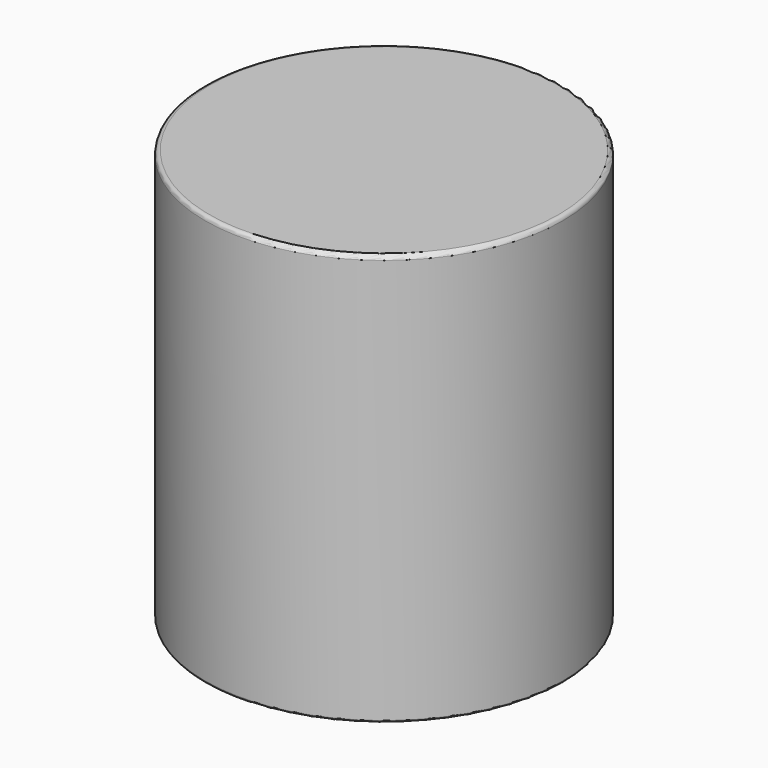
from build123d import *

# Parameters (mm, degrees)
F0_R     = 43.5
F0_R_2   = 42.5
F1_DEPTH = 100
F2_R     = 43.5
F3_DEPTH = 2
F4_R     = 1
F5_R     = 0.49999


# Not quite as in the source:
# - a fillet or chamfer is up to 0.001 mm smaller than in the source, because OpenCascade refuses the exact size


with BuildPart() as f1:
    # F0 (on Top) → F1 (new body)
    with BuildSketch(Plane.XY):
        Circle(F0_R)
        Circle(F0_R_2, mode=Mode.SUBTRACT)
    extrude(amount=F1_DEPTH)

    # F2 (on face) → F3 (join)
    with BuildSketch(Plane.XY.offset(100)):
        Circle(F2_R)
    extrude(amount=-F3_DEPTH)

    # F4
    f4_edges = [f1.edges().sort_by_distance(p)[0] for p in [
        (-43.5, 0, 100),
    ]]
    fillet(f4_edges, radius=F4_R)

    # F5 (radius 0.5 in the source; OpenCascade refuses exactly that, so slightly less here)
    f5_edges = [f1.edges().sort_by_distance(p)[0] for p in [
        (-43.5, 0, 0),
        (-42.5, 0, 0),
    ]]
    fillet(f5_edges, radius=F5_R)


solid = f1.part
